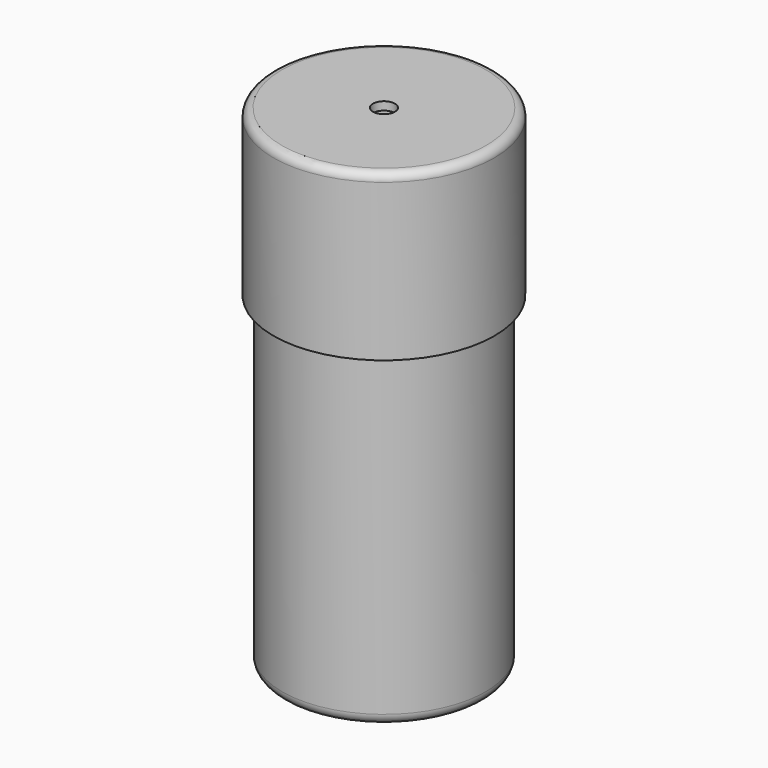
from build123d import *


# Not quite as in the source:
# - a fillet or chamfer that OpenCascade refuses, or shapes differently, is made with other operations: its cross-section is extruded or revolved along the edge and cut away or added


with BuildPart() as f1:
    # F0 (on Front) → F1 (revolve)
    with BuildSketch(Plane.XZ):
        Polygon((-2, 0), (-2, 1.5), (-17, 1.5), (-17, 88), (-18.5, 88), (-18.5, 0), align=None)
    revolve(axis=Axis((0, 0, 38.7278981507), (0, 0, 1)))

    # F2: fillet of radius 2 on 3 edges, made by hand

    # F2_s1 → F2_t2 (revolve)
    with BuildSketch(Plane.XZ):
        with BuildLine():
            ThreePointArc((-15, 1.5), (-16.4142135624, 2.0857864376), (-17, 3.5))
            Line((-17, 3.5), (-17, 1.5))
            Line((-17, 1.5), (-15, 1.5))
        make_face()
    revolve(axis=Axis((0, 0, 1.5), (0, 0, 1)))

    # F2_s3 → F2_t4 (revolve, cut)
    with BuildSketch(Plane.XZ):
        with BuildLine():
            ThreePointArc((-18.5, 86.0635083269), (-18.0811388301, 87.2882531983), (-17, 88))
            Line((-17, 88), (-18.5, 88))
            Line((-18.5, 88), (-18.5, 86.0635083269))
        make_face()
    revolve(axis=Axis((0, 0, 88), (0, 0, 1)), mode=Mode.SUBTRACT)

    # F2_s5 → F2_t6 (revolve, cut)
    with BuildSketch(Plane.XZ):
        with BuildLine():
            ThreePointArc((-16.5, 0), (-17.9142135624, 0.5857864376), (-18.5, 2))
            Line((-18.5, 2), (-18.5, 0))
            Line((-18.5, 0), (-16.5, 0))
        make_face()
    revolve(axis=Axis((0, 0, 0), (0, 0, 1)), mode=Mode.SUBTRACT)


with BuildPart() as f4:
    # F3 (on Front) → F4 (revolve)
    with BuildSketch(Plane.XZ):
        with BuildLine():
            Line((-20.0970838815, 88), (-20.0970838815, 59.5))
            Line((-20.0970838815, 59.5), (-19.5, 59.5))
            Line((-19.5, 59.5), (-18.75, 60.25))
            Line((-18.75, 60.25), (-18.75, 86.5))
            ThreePointArc((-18.75, 86.5), (-18.3106601718, 87.5606601718), (-17.25, 88))
            Line((-17.25, 88), (-2, 88))
            Line((-2, 88), (-2, 89.5))
            Line((-2, 89.5), (-18.5970838815, 89.5))
            ThreePointArc((-18.5970838815, 89.5), (-19.6577440533, 89.0606601718), (-20.0970838815, 88))
        make_face()
    revolve(axis=Axis((0, 0, 24.4026009697), (0, 0, 1)))


solid = Compound([f1.part, f4.part])
